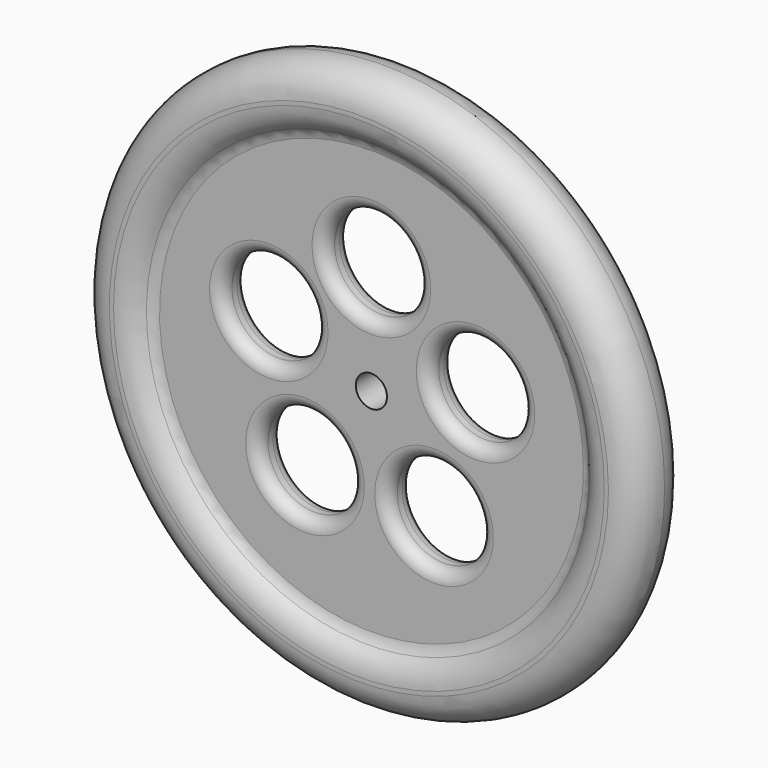
from build123d import *

# Parameters (mm, degrees)
F0_R     = 114.3
F0_R_2   = 88.9
F1_DEPTH = 12.7
F0_R_3   = 19.05
F0_R_4   = 6.35
F2_DEPTH = 6.35
F4_R     = 5.08
F5_R     = 5.08


# Not quite as in the source:
# - a fillet or chamfer that OpenCascade refuses, or shapes differently, is made with other operations: its cross-section is extruded or revolved along the edge and cut away or added


with BuildPart() as f1:
    # F0 (on Front) → F1 (new body, symmetric)
    with BuildSketch(Plane.XZ):
        Circle(F0_R)
        Circle(F0_R_2, mode=Mode.SUBTRACT)
    extrude(amount=F1_DEPTH, both=True)

    # F0 (on Front) → F2 (join, symmetric)
    with BuildSketch(Plane.XZ):
        Circle(F0_R_2)
        with Locations((-27.0594455194, -35.2645559759)):
            Circle(F0_R_3, mode=Mode.SUBTRACT)
        with Locations((25.4954725958, -36.4113083686)):
            Circle(F0_R_3, mode=Mode.SUBTRACT)
        with Locations((-41.7693369939, 15.2027953708)):
            Circle(F0_R_3, mode=Mode.SUBTRACT)
        Circle(F0_R_4, mode=Mode.SUBTRACT)
        with Locations((42.3927184608, 13.366372788)):
            Circle(F0_R_3, mode=Mode.SUBTRACT)
        with Locations((0, 44.45)):
            Circle(F0_R_3, mode=Mode.SUBTRACT)
    extrude(amount=F2_DEPTH, both=True)

    # F3: fillet of radius 12.7 on 4 edges, made by hand

    # F3_s1 → F3_t2 (revolve, cut)
    with BuildSketch(Plane.XY):
        with BuildLine():
            ThreePointArc((114.3, 0), (110.5802561211, -8.9802561211), (101.6, -12.7))
            Line((101.6, -12.7), (114.3, -12.7))
            Line((114.3, -12.7), (114.3, 0))
        make_face()
    revolve(axis=Axis((0, -12.7, 0), (0, -1, 0)), mode=Mode.SUBTRACT)

    # F3_s3 → F3_t4 (revolve, cut)
    with BuildSketch(Plane.XY):
        with BuildLine():
            ThreePointArc((114.3, 0), (110.5802561211, 8.9802561211), (101.6, 12.7))
            Line((101.6, 12.7), (114.3, 12.7))
            Line((114.3, 12.7), (114.3, 0))
        make_face()
    revolve(axis=Axis((0, 12.7, 0), (0, -1, 0)), mode=Mode.SUBTRACT)

    # F3_s5 → F3_t6 (revolve, cut)
    with BuildSketch(Plane.XY):
        with BuildLine():
            ThreePointArc((99.8985226281, 12.7), (93.5485226281, 10.9985226281), (88.9, 6.35))
            Line((88.9, 6.35), (88.9, 12.7))
            Line((88.9, 12.7), (99.8985226281, 12.7))
        make_face()
    revolve(axis=Axis((0, 12.7, 0), (0, -1, 0)), mode=Mode.SUBTRACT)

    # F3_s7 → F3_t8 (revolve, cut)
    with BuildSketch(Plane.XY):
        with BuildLine():
            ThreePointArc((99.8985226281, -12.7), (93.5485226281, -10.9985226281), (88.9, -6.35))
            Line((88.9, -6.35), (88.9, -12.7))
            Line((88.9, -12.7), (99.8985226281, -12.7))
        make_face()
    revolve(axis=Axis((0, -12.7, 0), (0, -1, 0)), mode=Mode.SUBTRACT)

    # F4
    f4_edges = [f1.edges().sort_by_distance(p)[0] for p in [
        (6.445473, -6.35, -36.411308),
        (6.445473, 6.35, -36.411308),
        (-46.109446, -6.35, -35.264556),
        (-46.109446, 6.35, -35.264556),
        (-60.819337, -6.35, 15.202795),
        (-60.819337, 6.35, 15.202795),
        (-19.05, -6.35, 44.45),
        (-19.05, 6.35, 44.45),
        (23.342718, 6.35, 13.366373),
        (23.342718, -6.35, 13.366373),
    ]]
    fillet(f4_edges, radius=F4_R)

    # F5
    f5_edges = [f1.edges().sort_by_distance(p)[0] for p in [
        (-88.9, -6.35, 0),
        (-88.9, 6.35, 0),
    ]]
    fillet(f5_edges, radius=F5_R)


solid = f1.part
